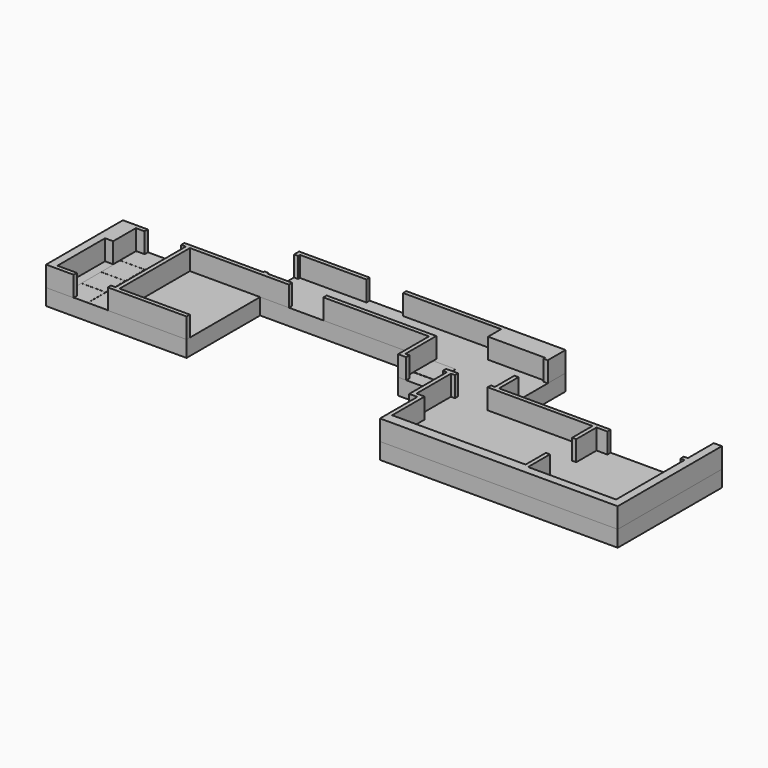
from build123d import *

# Parameters (mm, degrees)
F0_W     = 1730
F0_H     = 2165
F1_DEPTH = 400
F2_DEPTH = 500
F3_W     = 600
F3_H     = 600
F4_DEPTH = 6
F3_W_2   = 120.124710083
F3_H_2   = 103
F3_W_3   = 556.7045936584
F5_DEPTH = 6


with BuildPart() as f1:
    # F0 (on Top) → F1 (new body)
    with BuildSketch(Plane.XY):
        Polygon((0, 142.0842932612), (0, 2200), (-100, 2200), (-100, 2300), (-1900, 2300), (-1900, 2200), (-2168.751001358, 2200), (-2168.751001358, 1575), (-2268.751001358, 1575), (-2268.751001358, 2200), (-4650, 2200), (-4750, 2200), (-4850, 2200), (-4850, 2300), (-4750, 2300), (-4750, 2900), (-4650, 2900), (-4650, 3250), (-4650, 3800), (-4750, 3800), (-4750, 3850), (-6160, 3850), (-6160, 4250), (-8575, 4250), (-8575, 4350), (-9475, 4350), (-9475, 4250), (-11115, 4250), (-11115, 4195), (-11215, 4195), (-11215, 3285), (-11115, 3285), (-11115, 3250), (-10505.7045936584, 3250), (-10505.7045936584, 3150), (-9655.7045936584, 3150), (-9655.7045936584, 3250), (-7055.7045936584, 3250), (-6955.7045936584, 3250), (-6955.7045936584, 3150), (-6955.7045936584, 2300), (-6855.7045936584, 2300), (-6855.7045936584, 2200), (-5955.7045936584, 2200), (-5955.7045936584, 2300), (-5655.7045936584, 2300), (-5655.7045936584, 2200), (-5755.7045936584, 2200), (-5755.7045936584, 1142.0842932612), (-5555.7045936584, 1142.0842932612), (-5555.7045936584, 142.0842932612), (-2268.751001358, 142.0842932612), (-2268.751001358, 767.0842932612), (-2168.751001358, 767.0842932612), (-2168.751001358, 142.0842932612), (-2168.751001358, 92.0842932612), (0, 92.0842932612), align=None)
        Polygon((-100, 2200), (0, 2200), (0, 142.0842932612), (200, 142.0842932612), (200, 3100), (0, 3100), (0, 2300), (-100, 2300), align=None)
        Polygon((200, 142.0842932612), (0, 142.0842932612), (0, 92.0842932612), (-2168.751001358, 92.0842932612), (-2168.751001358, 142.0842932612), (-2168.751001358, 767.0842932612), (-2268.751001358, 767.0842932612), (-2268.751001358, 142.0842932612), (-5555.7045936584, 142.0842932612), (-5555.7045936584, 1142.0842932612), (-5755.7045936584, 1142.0842932612), (-5755.7045936584, 2200), (-5655.7045936584, 2200), (-5655.7045936584, 2300), (-5955.7045936584, 2300), (-5955.7045936584, 2200), (-5855.7045936584, 2200), (-5855.7045936584, 1042.0842932612), (-5655.7045936584, 1042.0842932612), (-5655.7045936584, -107.9157067388), (200, -107.9157067388), (200, 0), align=None)
        Polygon((-1900, 2200), (-1900, 2300), (-4650, 2300), (-4650, 2900), (-4750, 2900), (-4750, 2300), (-4850, 2300), (-4850, 2200), (-4750, 2200), (-4650, 2200), (-2268.751001358, 2200), (-2268.751001358, 1575), (-2168.751001358, 1575), (-2168.751001358, 2200), align=None)
        Polygon((-4750, 3800), (-4650, 3800), (-4650, 4250), (-4650, 4350), (-4750, 4350), (-8575, 4350), (-8575, 4250), (-6160, 4250), (-6160, 3850), (-4750, 3850), align=None)
        Polygon((-7055.7045936584, 2200), (-6855.7045936584, 2200), (-6855.7045936584, 2300), (-6955.7045936584, 2300), (-6955.7045936584, 3150), (-6955.7045936584, 3250), (-7055.7045936584, 3250), (-9655.7045936584, 3250), (-9655.7045936584, 3150), (-7055.7045936584, 3150), align=None)
        Polygon((-9475, 4250), (-9475, 4350), (-11115, 4350), (-11215, 4350), (-11215, 4195), (-11115, 4195), (-11115, 4250), align=None)
        Polygon((-11215, 3150), (-10505.7045936584, 3150), (-10505.7045936584, 3250), (-11115, 3250), (-11115, 3285), (-11215, 3285), (-11215, 3250), align=None)
        Polygon((-12945, 3150), (-11215, 3150), (-11215, 3250), (-12945, 3250), (-13160, 3250), (-13160, 3150), (-13045, 3150), (-13045, 985), (-12945, 985), align=None)
        with Locations((-12080, 2067.5)):
            Rectangle(F0_W, F0_H)
        Polygon((-11215, 885), (-11215, 985), (-12945, 985), (-13045, 985), (-13155, 985), (-13155, 885), align=None)
        Polygon((-13995, 885), (-13155, 885), (-13155, 985), (-13045, 985), (-13045, 3150), (-13160, 3150), (-13160, 3250), (-14060, 3250), (-14060, 3150), (-14275, 3150), (-14275, 2450), (-14475, 2450), (-14475, 985), (-13995, 985), align=None)
        Polygon((-14475, 885), (-13995, 885), (-13995, 985), (-14475, 985), (-14475, 2450), (-14275, 2450), (-14275, 3150), (-14060, 3150), (-14060, 3250), (-14675, 3250), (-14675, 985), (-14675, 885), align=None)
    extrude(amount=-F1_DEPTH)


with BuildPart() as f2:
    # F0 (on Top) → F2 (new body)
    with BuildSketch(Plane.XY):
        Polygon((-9475, 4250), (-9475, 4350), (-11115, 4350), (-11215, 4350), (-11215, 4195), (-11115, 4195), (-11115, 4250), align=None)
    extrude(amount=F2_DEPTH)


with BuildPart() as f2b:
    # F0 (on Top) → F2, piece 2 (new body)
    with BuildSketch(Plane.XY):
        Polygon((-4750, 3800), (-4650, 3800), (-4650, 4250), (-4650, 4350), (-4750, 4350), (-8575, 4350), (-8575, 4250), (-6160, 4250), (-6160, 3850), (-4750, 3850), align=None)
    extrude(amount=F2_DEPTH)


with BuildPart() as f2c:
    # F0 (on Top) → F2, piece 3 (new body)
    with BuildSketch(Plane.XY):
        Polygon((-11215, 3150), (-10505.7045936584, 3150), (-10505.7045936584, 3250), (-11115, 3250), (-11115, 3285), (-11215, 3285), (-11215, 3250), align=None)
        Polygon((-12945, 3150), (-11215, 3150), (-11215, 3250), (-12945, 3250), (-13160, 3250), (-13160, 3150), (-13045, 3150), (-13045, 985), (-12945, 985), align=None)
        Polygon((-11215, 885), (-11215, 985), (-12945, 985), (-13045, 985), (-13155, 985), (-13155, 885), align=None)
    extrude(amount=F2_DEPTH)


with BuildPart() as f2d:
    # F0 (on Top) → F2, piece 4 (new body)
    with BuildSketch(Plane.XY):
        Polygon((-14475, 885), (-13995, 885), (-13995, 985), (-14475, 985), (-14475, 2450), (-14275, 2450), (-14275, 3150), (-14060, 3150), (-14060, 3250), (-14675, 3250), (-14675, 985), (-14675, 885), align=None)
    extrude(amount=F2_DEPTH)


with BuildPart() as f2e:
    # F0 (on Top) → F2, piece 5 (new body)
    with BuildSketch(Plane.XY):
        Polygon((200, 142.0842932612), (0, 142.0842932612), (0, 92.0842932612), (-2168.751001358, 92.0842932612), (-2168.751001358, 142.0842932612), (-2168.751001358, 767.0842932612), (-2268.751001358, 767.0842932612), (-2268.751001358, 142.0842932612), (-5555.7045936584, 142.0842932612), (-5555.7045936584, 1142.0842932612), (-5755.7045936584, 1142.0842932612), (-5755.7045936584, 2200), (-5655.7045936584, 2200), (-5655.7045936584, 2300), (-5955.7045936584, 2300), (-5955.7045936584, 2200), (-5855.7045936584, 2200), (-5855.7045936584, 1042.0842932612), (-5655.7045936584, 1042.0842932612), (-5655.7045936584, -107.9157067388), (200, -107.9157067388), (200, 0), align=None)
        Polygon((-100, 2200), (0, 2200), (0, 142.0842932612), (200, 142.0842932612), (200, 3100), (0, 3100), (0, 2300), (-100, 2300), align=None)
    extrude(amount=F2_DEPTH)


with BuildPart() as f2f:
    # F0 (on Top) → F2, piece 6 (new body)
    with BuildSketch(Plane.XY):
        Polygon((-1900, 2200), (-1900, 2300), (-4650, 2300), (-4650, 2900), (-4750, 2900), (-4750, 2300), (-4850, 2300), (-4850, 2200), (-4750, 2200), (-4650, 2200), (-2268.751001358, 2200), (-2268.751001358, 1575), (-2168.751001358, 1575), (-2168.751001358, 2200), align=None)
    extrude(amount=F2_DEPTH)


with BuildPart() as f2g:
    # F0 (on Top) → F2, piece 7 (new body)
    with BuildSketch(Plane.XY):
        Polygon((-7055.7045936584, 2200), (-6855.7045936584, 2200), (-6855.7045936584, 2300), (-6955.7045936584, 2300), (-6955.7045936584, 3150), (-6955.7045936584, 3250), (-7055.7045936584, 3250), (-9655.7045936584, 3250), (-9655.7045936584, 3150), (-7055.7045936584, 3150), align=None)
    extrude(amount=F2_DEPTH)


with BuildPart() as f4:
    # F3 (on face) → F4 (new body)
    with BuildSketch(Plane.XY):
        with Locations((-13346.5, 2347)):
            Rectangle(F3_W, F3_H)
    extrude(amount=F4_DEPTH)


with BuildPart() as f4b:
    # F3 (on face) → F4, piece 2 (new body)
    with BuildSketch(Plane.XY):
        with Locations((-13949.5, 2347)):
            Rectangle(F3_W, F3_H)
    extrude(amount=F4_DEPTH)


with BuildPart() as f4c:
    # F3 (on face) → F4, piece 3 (new body)
    with BuildSketch(Plane.XY):
        Polygon((-13163, 3250), (-13646.5, 3250), (-13646.5, 2650), (-13042.875289917, 2650), (-13042.875289917, 3147), (-13163, 3147), align=None)
        Polygon((-13646.5, 2650), (-13646.5, 3250), (-14057, 3250), (-14057, 3147), (-14249.5, 3147), (-14249.5, 2650), align=None)
        with Locations((-13102.9376449585, 3198.5)):
            Rectangle(F3_W_2, F3_H_2)
    extrude(amount=F4_DEPTH)


with BuildPart() as f4d:
    # F3 (on face) → F4, piece 4 (new body)
    with BuildSketch(Plane.XY):
        Polygon((-13992, 988), (-13992, 885), (-13649.5, 885), (-13649.5, 1441), (-14249.5, 1441), (-14249.5, 988), align=None)
    extrude(amount=F4_DEPTH)


with BuildPart() as f4e:
    # F3 (on face) → F4, piece 5 (new body)
    with BuildSketch(Plane.XY):
        with Locations((-13949.5, 1744)):
            Rectangle(F3_W, F3_H)
    extrude(amount=F4_DEPTH)


with BuildPart() as f4f:
    # F3 (on face) → F4, piece 6 (new body)
    with BuildSketch(Plane.XY):
        with Locations((-13346.5, 1744)):
            Rectangle(F3_W, F3_H)
    extrude(amount=F4_DEPTH)


with BuildPart() as f4g:
    # F3 (on face) → F4, piece 7 (new body)
    with BuildSketch(Plane.XY):
        with Locations((-6672.3522968292, 2845.5)):
            Rectangle(F3_W_3, F3_H)
    extrude(amount=F4_DEPTH)


with BuildPart() as f5:
    # F3 (on face) → F5 (new body)
    with BuildSketch(Plane.XY):
        Polygon((-13646.5, 1441), (-13646.5, 885), (-13158, 885), (-13158, 988), (-13046.5, 988), (-13046.5, 1441), align=None)
    extrude(amount=F5_DEPTH)


solid = Compound([f1.part, f2.part, f2b.part, f2c.part, f2d.part, f2e.part, f2f.part, f2g.part, f4.part, f4b.part, f4c.part, f4d.part, f4e.part, f4f.part, f4g.part, f5.part])
